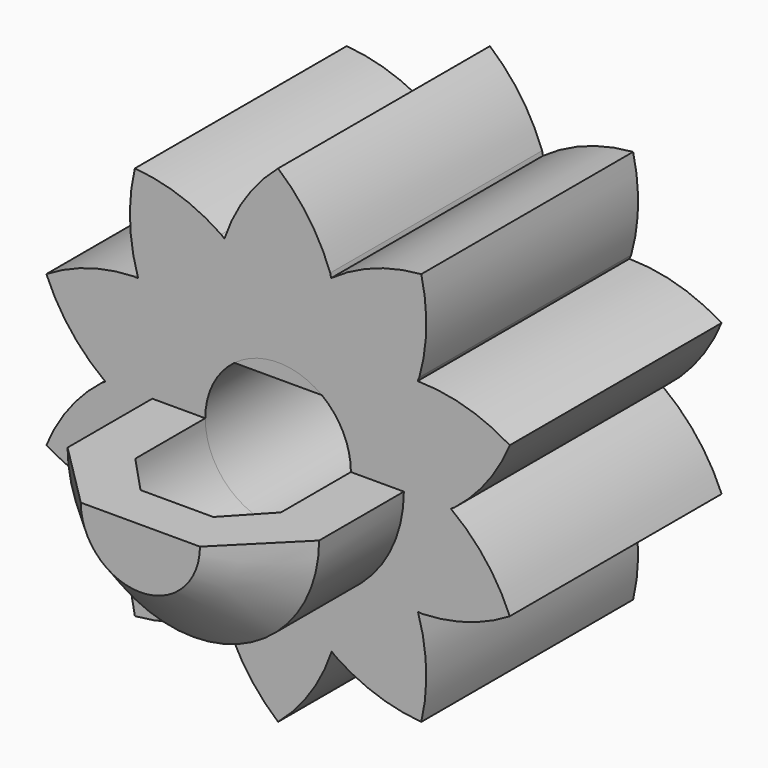
from build123d import *
from build123d import SkipClean  # not in build123d's __all__

# Parameters (mm, degrees)
F0_W            = 6.5
F0_H            = 10
F3_DEPTH        = 25
F5_DEPTH        = 10
F5_COPIES_COUNT = 10
F7_DEPTH        = 6.5
F9_SIZE         = 2.5


# Not quite as in the source:
# - a pattern or mirror of a feature is missing from the dataset's text; its kind, count and spacing are read off the source's solid
# - a feature names something its author has since deleted; it is built from what else it names


with BuildPart() as f1:
    # F0 (on Top) → F1 (revolve)
    with BuildSketch(Plane.XY):
        with Locations((-3.25, 5)):
            Rectangle(F0_W, F0_H)
    revolve(axis=Axis((0, 5, 0), (0, 1, 0)))

    # F2 (on face) → F3 (cut)
    with BuildSketch(Plane(origin=(0, 10, 0), x_dir=(-1, 0, 0), z_dir=(0, 1, 0))):
        with BuildLine():
            Line((1.65, 2.2), (-1.65, 2.2))
            ThreePointArc((-1.65, 2.2), (0, -2.75), (1.65, 2.2))
        make_face()
    extrude(amount=-F3_DEPTH, mode=Mode.SUBTRACT)

    # F4 (on face) → F5 (join)
    with BuildSketch(Plane(origin=(0, 10, 0), x_dir=(-1, 0, 0), z_dir=(0, 1, 0))):
        with BuildLine():
            ThreePointArc((-2.0086104634, 6.1818673559), (0.0140777422, 6.4999847551), (2.0353690139, 6.1731088584))
            ThreePointArc((2.0353690139, 6.1731088584), (1.2263837508, 7.8268898276), (0, 9.2))
            ThreePointArc((0, 9.2), (-1.1693294851, 7.9103781541), (-1.9692767773, 6.3642409415))
            ThreePointArc((-1.9692767773, 6.3642409415), (-1.9898456325, 6.2732486915), (-2.0086104634, 6.1818673559))
        make_face()
    f5 = extrude(amount=-F5_DEPTH)

    # F5_copies: F5 ×10 about axis
    f5_copies_axis = Axis((0, 0, 0), (0, 1, 0))
    for i in range(1, F5_COPIES_COUNT):
        add(f5.rotate(f5_copies_axis, i * 360 / F5_COPIES_COUNT), clean=False)

    # F6 (on face) → F7 (join)
    with BuildSketch(Plane.XZ):
        with BuildLine():
            Line((-2.75, 0), (-4.75, 0))
            ThreePointArc((-4.75, 0), (0, -4.75), (4.75, 0))
            Line((4.75, 0), (2.75, 0))
            ThreePointArc((2.75, 0), (0, -2.75), (-2.75, 0))
        make_face()
        with BuildLine():
            Line((2.75, 0), (-2.75, 0))
            ThreePointArc((-2.75, 0), (0, -2.75), (2.75, 0))
        make_face()
    extrude(amount=F7_DEPTH)

    # F9
    f9_edges = [f1.edges().sort_by_distance(p)[0] for p in [
        (0, -6.5, -4.75),
    ]]
    chamfer(f9_edges, length=F9_SIZE)

    # F8 (on face) → F10 (revolve, cut)
    with BuildSketch(Plane.XY):
        Polygon((0, -1.3273195364), (0, 0), (-2.75, 0), (-2.75, -3.3025264561), (-1.375, -4.775), (0, -4.775), (0, -3.3025264561), (0, -1.8300529122), align=None)
    with SkipClean():  # cleaning this boolean's faces spoils the solid; the shape is the same uncleaned
        revolve(axis=Axis((0, -3.3025264561, 0), (0, -1, 0)), mode=Mode.SUBTRACT)


solid = f1.part
